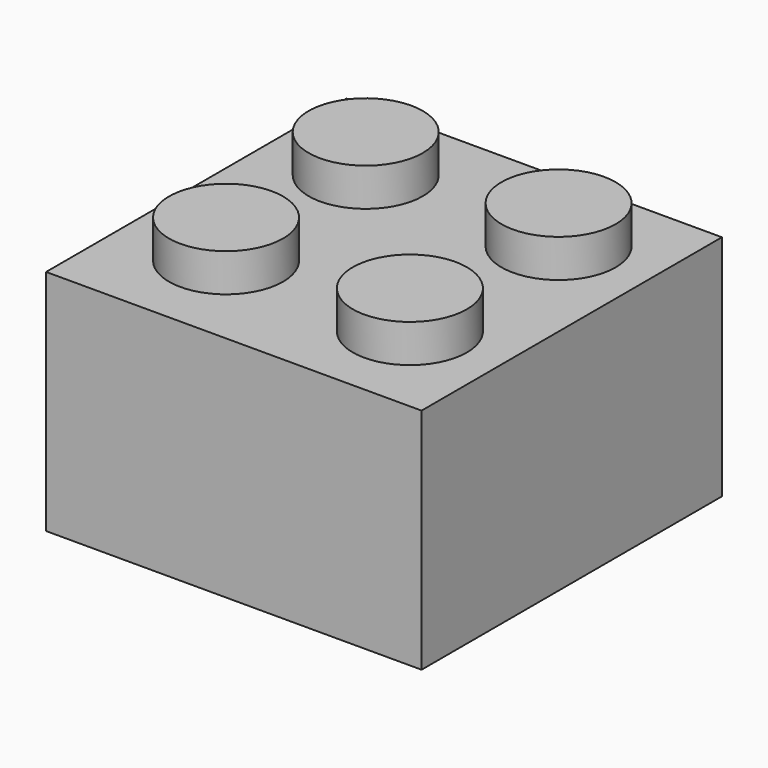
from build123d import *

# Parameters (mm, degrees)
F0_W          = 15.8
F0_H          = 15.8
F1_DEPTH      = 9.6
F4_R          = 2.4
F6_DEPTH      = 1.6
F5_R          = 2.4
F7_DEPTH      = 1.6
F3_R          = 2.4
F8_DEPTH      = 1.6
F2_R          = 2.4
F9_DEPTH      = 1.6
F10_T         = -1
F11_R         = 4.255
F12_DEPTH     = 8.13
F13_T         = 1
F13_T3_DEPTH  = 10.6
F13_T5_DEPTH  = 15.8
F13_T7_DEPTH  = 15.8
F13_T18_ANGLE = 35.7281901551
F13_T20_ANGLE = 210.9230732258
F13_T22_ANGLE = 74.818128958
F13_T24_ANGLE = 41.9866867229
F13_T28_ANGLE = 82.2344866513


# Not quite as in the source:
# - a shell that OpenCascade refuses in one call is made with other operations: the cavity is built on its own and cut out


with BuildPart() as f1:
    # F0 (on Top) → F1 (new body)
    with BuildSketch(Plane.XY):
        Rectangle(F0_W, F0_H)
    extrude(amount=-F1_DEPTH)

    # F4 (on face) → F6 (join)
    with BuildSketch(Plane.XY):
        with Locations((-3.7834926043, -3.5802270286)):
            Circle(F4_R)
    extrude(amount=F6_DEPTH)

    # F5 (on face) → F7 (join)
    with BuildSketch(Plane.XY):
        with Locations((4.0790652856, -3.737478517)):
            Circle(F5_R)
    extrude(amount=F7_DEPTH)

    # F3 (on face) → F8 (join)
    with BuildSketch(Plane.XY):
        with Locations((4.1130073369, 4.042240791)):
            Circle(F3_R)
    extrude(amount=F8_DEPTH)

    # F2 (on face) + F3 (on face) → F9 (join)
    with BuildSketch(Plane.XY):
        with Locations((-4.0000770241, 4.039389547)):
            Circle(F2_R)
    with BuildSketch(Plane.XY):
        with Locations((4.1130073369, 4.042240791)):
            Circle(F3_R)
    extrude(amount=F9_DEPTH)

    # F10
    f10_openings = [f1.faces().sort_by_distance(p)[0] for p in [
        (0, 0, -9.6),
    ]]
    offset(amount=F10_T, openings=f10_openings, kind=Kind.INTERSECTION)

    # F11 (on face) → F12 (join)
    with BuildSketch(Plane(origin=(0, 0, -1), x_dir=(1, 0, 0), z_dir=(0, 0, -1))):
        Circle(F11_R)
    extrude(amount=F12_DEPTH)

    # F13: shell of thickness 1, made by hand


with BuildPart() as f13_core1:
    # F13_t2: copy of F1
    add(f1.part)

    # the walls: a layer under each face that stays
    f13_faces = [f13_core1.faces().sort_by_distance(p)[0] for p in [
        (7.9, 0, -4.8),
        (0, -7.9, -4.8),
        (0, 7.9, -4.8),
        (0, 0, 0),
        (-7.3733333333, -7.3733333333, -9.6),
        (-7.9, 0, -4.8),
        (-6.1834926043, -3.5802270286, 0.8),
        (1.6790652856, -3.737478517, 0.8),
        (-6.4000770241, 4.039389547, 0.8),
        (1.7130073369, 4.042240791, 0.8),
        (6.9, 0, -5.3),
        (0, -6.9, -5.3),
        (-6.9, 0, -5.3),
        (0, 6.9, -5.3),
        (-3.7834926043, -3.5802270286, 1.6),
        (4.0790652856, -3.737478517, 1.6),
        (-4.0000770241, 4.039389547, 1.6),
        (4.1130073369, 4.042240791, 1.6),
        (-4.6, 0, -1),
        (2.6790652856, -3.737478517, -0.2),
        (-4.255, 0, -5.065),
        (-5.1834926043, -3.5802270286, -0.2),
        (-5.4000770241, 4.039389547, -0.2),
        (2.7130073369, 4.042240791, -0.2),
        (3.1153566982, -2.8544722668, -1),
        (4.0790652856, -3.737478517, 0.6),
        (-3.0174039644, -2.8552959816, -1),
        (-3.7834926043, -3.5802270286, 0.6),
        (-4.0000770241, 4.039389547, 0.6),
        (4.1130073369, 4.042240791, 0.6),
    ]]
    thicken(f13_faces, amount=-F13_T, mode=Mode.SUBTRACT)

    # F13_s4 → F13_t3 (cut)
    with BuildSketch(Plane.XY.offset(-10.6)):
        Polygon((6.89, -6.89), (7.9, -6.9), (7.9, -7.9), (6.9, -7.9), align=None)
        Polygon((6.89, 6.89), (7.9, 6.9), (7.9, 7.9), (6.9, 7.9), align=None)
        Polygon((-6.89, -6.89), (-6.9, -7.9), (-7.9, -7.9), (-7.9, -6.9), align=None)
        Polygon((-6.89, 6.89), (-7.9, 6.9), (-7.9, 7.9), (-6.9, 7.9), align=None)
    extrude(amount=F13_T3_DEPTH, mode=Mode.SUBTRACT)

    # F13_s6 → F13_t5 (cut)
    with BuildSketch(Plane.XZ.offset(-7.9)):
        Polygon((6.89, -1.01), (7.9, -1), (7.9, 0), (6.9, 0), align=None)
        Polygon((-6.89, -1.01), (-7.9, -1), (-7.9, 0), (-6.9, 0), align=None)
    extrude(amount=F13_T5_DEPTH, mode=Mode.SUBTRACT)

    # F13_s8 → F13_t7 (cut)
    with BuildSketch(Plane.YZ.offset(-7.9)):
        Polygon((-6.89, -1.01), (-7.9, -1), (-7.9, 0), (-6.9, 0), align=None)
        Polygon((6.89, -1.01), (7.9, -1), (7.9, 0), (6.9, 0), align=None)
    extrude(amount=F13_T7_DEPTH, mode=Mode.SUBTRACT)

    # F13_s9 → F13_t10 (revolve, cut)
    with BuildSketch(Plane.XZ.offset(3.5802270286)):
        Polygon((-1.3734926043, 0.01), (-1.3834926043, -1), (-2.3834926043, -1), (-2.3834926043, 0), align=None)
    revolve(axis=Axis((-3.7834926043, -3.5802270286, 0), (0, 0, 1)), mode=Mode.SUBTRACT)

    # F13_s11 → F13_t12 (revolve, cut)
    with BuildSketch(Plane.XZ.offset(3.737478517)):
        Polygon((6.4890652856, 0.01), (6.4790652856, -1), (5.4790652856, -1), (5.4790652856, 0), align=None)
    revolve(axis=Axis((4.0790652856, -3.737478517, 0), (0, 0, 1)), mode=Mode.SUBTRACT)

    # F13_s13 → F13_t14 (revolve, cut)
    with BuildSketch(Plane.XZ.offset(-4.039389547)):
        Polygon((-1.5900770241, 0.01), (-1.6000770241, -1), (-2.6000770241, -1), (-2.6000770241, 0), align=None)
    revolve(axis=Axis((-4.0000770241, 4.039389547, 0), (0, 0, 1)), mode=Mode.SUBTRACT)

    # F13_s15 → F13_t16 (revolve, cut)
    with BuildSketch(Plane.XZ.offset(-4.042240791)):
        Polygon((6.5230073369, 0.01), (6.5130073369, -1), (5.5130073369, -1), (5.5130073369, 0), align=None)
    revolve(axis=Axis((4.1130073369, 4.042240791, 0), (0, 0, 1)), mode=Mode.SUBTRACT)

    # F13_s17 → F13_t18 (revolve, cut)
    with BuildSketch(Plane.XZ):
        Polygon((4.265, -1.01), (4.255, 0), (3.255, 0), (3.255, -1), align=None)
    revolve(axis=Axis((0, 0, -1), (0, 0, -1)), revolution_arc=F13_T18_ANGLE, mode=Mode.SUBTRACT)

    # F13_s19 → F13_t20 (revolve, cut)
    with BuildSketch(Plane(origin=(0, 0, 0), x_dir=(0, 0, 1), z_dir=(0.5138867564, -0.8578580312, 0))):
        Polygon((-1.01, 4.265), (0, 4.255), (0, 3.255), (-1, 3.255), align=None)
    revolve(axis=Axis((0, 0, -1), (0, 0, -1)), revolution_arc=F13_T20_ANGLE, mode=Mode.SUBTRACT)

    # F13_s21 → F13_t22 (revolve, cut)
    with BuildSketch(Plane(origin=(0, 0, 0), x_dir=(0, 0, 1), z_dir=(0.7577618984, 0.6525311528, 0))):
        Polygon((-1.01, 4.265), (0, 4.255), (0, 3.255), (-1, 3.255), align=None)
    revolve(axis=Axis((0, 0, -1), (0, 0, -1)), revolution_arc=F13_T22_ANGLE, mode=Mode.SUBTRACT)

    # F13_s23 → F13_t24 (revolve, cut)
    with BuildSketch(Plane(origin=(-0.7265604619, -1.8440663308, 0), x_dir=(0, 0, 1), z_dir=(-0.3665725996, -0.9303894503, 0))):
        Polygon((-0.99, -3.7751765248), (-1, -2.7651765248), (-2, -2.7651765248), (-2, -3.7651765248), align=None)
    revolve(axis=Axis((4.0790652856, -3.737478517, -1), (0, 0, -1)), revolution_arc=F13_T24_ANGLE, mode=Mode.SUBTRACT)

    # F13_s25 → F13_t26 (revolve, cut)
    with BuildSketch(Plane.XZ.offset(3.737478517)):
        Polygon((5.4690652856, 0.59), (6.4790652856, 0.6), (6.4790652856, 1.6), (5.4790652856, 1.6), align=None)
    revolve(axis=Axis((4.0790652856, -3.737478517, 0.6), (0, 0, -1)), mode=Mode.SUBTRACT)

    # F13_s27 → F13_t28 (revolve, cut)
    with BuildSketch(Plane(origin=(-3.4098320419, 0.3261629687, 0), x_dir=(0, 0, 1), z_dir=(-0.9954563431, 0.0952190583, 0))):
        Polygon((-0.99, -2.5342203081), (-1, -1.5242203081), (-2, -1.5242203081), (-2, -2.5242203081), align=None)
    revolve(axis=Axis((-3.7834926043, -3.5802270286, -1), (0, 0, -1)), revolution_arc=F13_T28_ANGLE, mode=Mode.SUBTRACT)

    # F13_s29 → F13_t30 (revolve, cut)
    with BuildSketch(Plane.XZ.offset(3.5802270286)):
        Polygon((-2.3934926043, 0.59), (-1.3834926043, 0.6), (-1.3834926043, 1.6), (-2.3834926043, 1.6), align=None)
    revolve(axis=Axis((-3.7834926043, -3.5802270286, 0.6), (0, 0, -1)), mode=Mode.SUBTRACT)

    # F13_s31 → F13_t32 (revolve, cut)
    with BuildSketch(Plane.XZ.offset(-4.039389547)):
        Polygon((-2.6100770241, 0.59), (-1.6000770241, 0.6), (-1.6000770241, 1.6), (-2.6000770241, 1.6), align=None)
    revolve(axis=Axis((-4.0000770241, 4.039389547, 0.6), (0, 0, -1)), mode=Mode.SUBTRACT)

    # F13_s33 → F13_t34 (revolve, cut)
    with BuildSketch(Plane.XZ.offset(-4.042240791)):
        Polygon((5.5030073369, 0.59), (6.5130073369, 0.6), (6.5130073369, 1.6), (5.5130073369, 1.6), align=None)
    revolve(axis=Axis((4.1130073369, 4.042240791, 0.6), (0, 0, -1)), mode=Mode.SUBTRACT)


with BuildPart() as f1_1:
    add(f1.part)

    # what is left inside the walls is the cavity
    f13_cavity = [f13_core1.part.solids().sort_by_distance(p)[0] for p in [
        (-3.245, 0, -6.42),
    ]]
    add(f13_cavity, mode=Mode.SUBTRACT)


solid = f1_1.part
